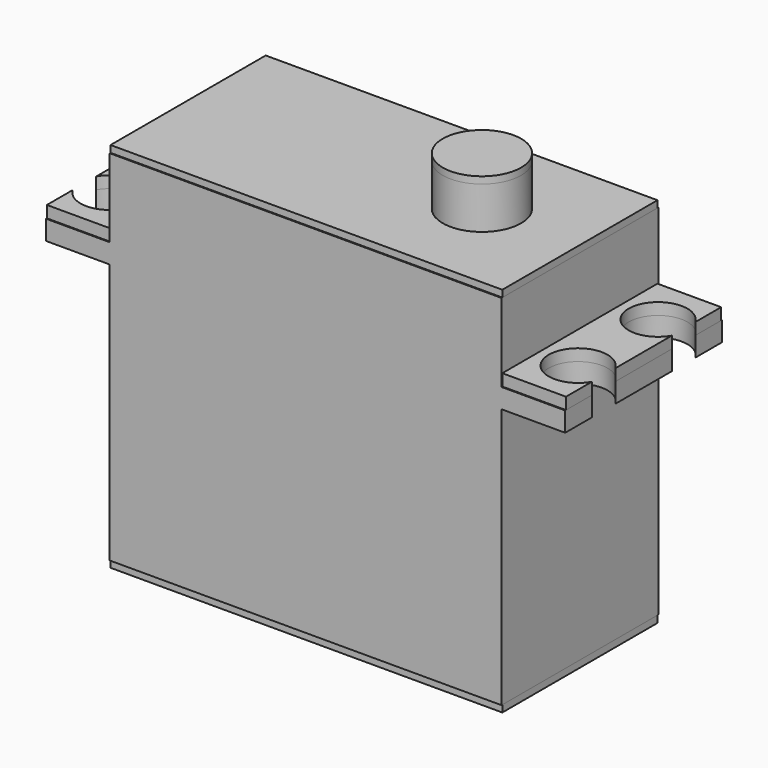
from build123d import *

# Parameters (mm, degrees)
F2_DEPTH = 9.9
F3_DEPTH = 10
F4_R     = 4
F5_DEPTH = 5
F6_R     = 4
F7_DEPTH = 5
F9_D     = 6
F9_2_D   = 6


with BuildPart() as f2:
    # F1 (on Front) → F2 (new body, symmetric)
    with BuildSketch(Plane.XZ):
        Polygon((-20, -19), (20, -19), (20, 9), (26.5, 9), (26.5, 11.5), (20, 11.5), (20, 19), (-20, 19), (-20, 11.5), (-26.5, 11.5), (-26.5, 9), (-20, 9), align=None)
    extrude(amount=F2_DEPTH, both=True)

    # F4 (on face) → F5 (join)
    with BuildSketch(Plane.XY.offset(19)):
        with Locations((10, 0)):
            Circle(F4_R)
    extrude(amount=F5_DEPTH)

    # F9 (through all)
    with Locations(Plane(origin=(0, 0, 0), x_dir=(1, 0, 0), z_dir=(0, 0, -1))):
        with Locations((-23.9, 5.1), (23.9, 5.1), (23.9, -5.1), (-23.9, -5.1)):
            Hole(F9_D / 2)


with BuildPart() as f3:
    # F0 (on Front) → F3 (new body, symmetric)
    with BuildSketch(Plane.XZ):
        Polygon((-20, -18.3), (20, -18.3), (20, 8.3), (26.5, 8.3), (26.5, 10.3), (20, 10.3), (20, 18.3), (-20, 18.3), (-20, 10.3), (-26.5, 10.3), (-26.5, 8.3), (-20, 8.3), align=None)
    extrude(amount=F3_DEPTH, both=True)

    # F6 (on face) → F7 (join)
    with BuildSketch(Plane.XY.offset(18.3)):
        with Locations((10, 0)):
            Circle(F6_R)
    extrude(amount=F7_DEPTH)

    # F9#2 (through all)
    with Locations(Plane(origin=(0, 0, 0), x_dir=(1, 0, 0), z_dir=(0, 0, -1))):
        with Locations((-23.9, 5.1), (23.9, 5.1), (23.9, -5.1), (-23.9, -5.1)):
            Hole(F9_2_D / 2)


solid = Compound([f2.part, f3.part])
